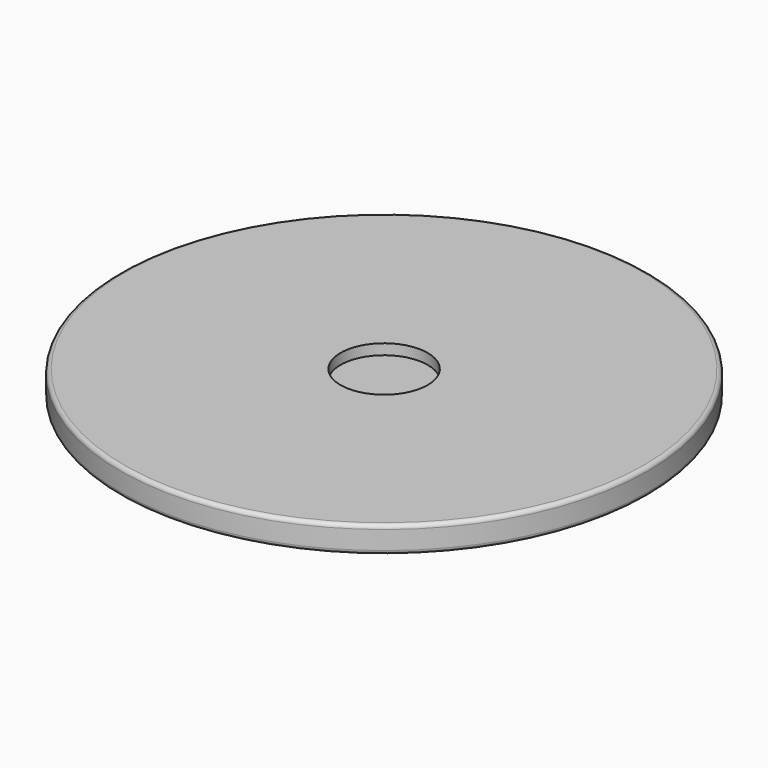
from build123d import *

# Parameters (mm, degrees)
F0_R     = 10
F1_DEPTH = 1
F2_R     = 0.15
F3_R     = 1.65
F4_DEPTH = 0.4


# Not quite as in the source:
# - a feature names something its author has since deleted; it is built from what else it names


with BuildPart() as f1:
    # F0 (on Top) → F1 (new body)
    with BuildSketch(Plane.XY):
        Circle(F0_R)
    extrude(amount=F1_DEPTH)

    # F2
    f2_edges = [f1.edges().sort_by_distance(p)[0] for p in [
        (-10, 0, 1),
        (-10, 0, 0),
    ]]
    fillet(f2_edges, radius=F2_R)

    # F3 (on face) → F4 (cut)
    with BuildSketch(Plane.XY.offset(1)):
        Circle(F3_R)
    extrude(amount=-F4_DEPTH, mode=Mode.SUBTRACT)


solid = f1.part
